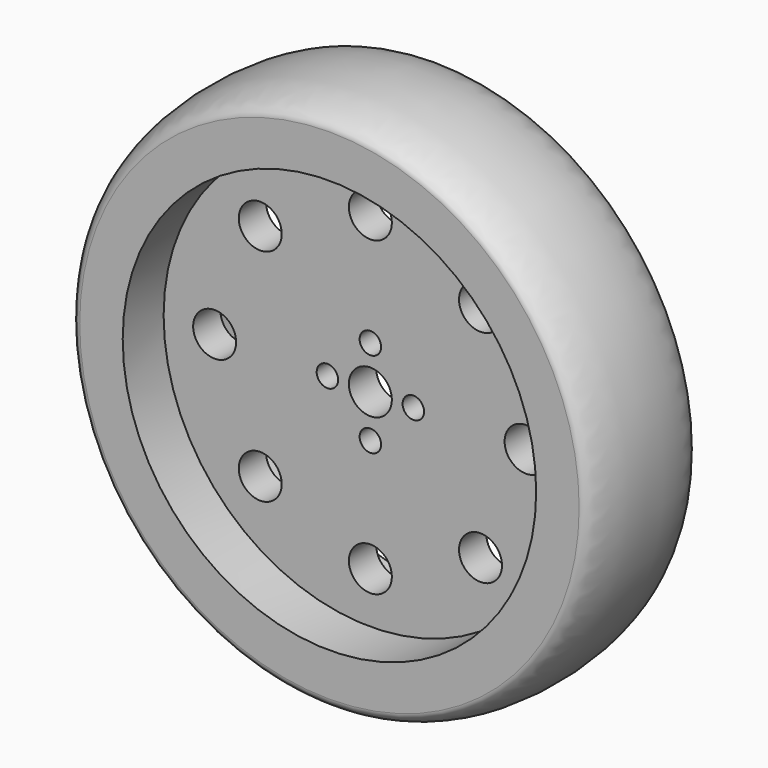
from build123d import *

# Parameters (mm, degrees)
F2_R     = 46.5
F2_R_2   = 38.5
F3_DEPTH = 12.7
F2_R_3   = 4
F2_R_4   = 2
F4_DEPTH = 3.175


# Not quite as in the source:
# - a length typed as a fraction of an inch, garbled in the dataset ("3 / 203.2 mm" for 3/8 in), is restored


with BuildPart() as f1:
    # F0 (on Right) → F1 (revolve)
    with BuildSketch(Plane.YZ):
        with BuildLine():
            Line((-12.7, 46.5), (12.7, 46.5))
            add(Edge.make_bspline(
                [(12.7, 46.5), (12.7, 50.2635093224), (0, 50.2635093224), (-12.7, 50.2635093224), (-12.7, 46.5)],
                knots=[0, 0, 0, 1.5707963268, 1.5707963268, 3.1415926536, 3.1415926536, 3.1415926536], degree=2, weights=[1, 0.7071067812, 1, 0.7071067812, 1]))
        make_face()
    revolve(axis=Axis((0, 0, 0), (0, 1, 0)))

    # F2 (on Front) → F3 (join, symmetric)
    with BuildSketch(Plane.XZ):
        Circle(F2_R)
        Circle(F2_R_2, mode=Mode.SUBTRACT)
    extrude(amount=F3_DEPTH, both=True)

    # F2 (on Front) → F4 (join, symmetric)
    with BuildSketch(Plane.XZ):
        Circle(F2_R_2)
        with Locations((-20.5060966544, -20.5060966544)):
            Circle(F2_R_3, mode=Mode.SUBTRACT)
        with Locations((0, -29)):
            Circle(F2_R_3, mode=Mode.SUBTRACT)
        with Locations((20.5060966544, -20.5060966544)):
            Circle(F2_R_3, mode=Mode.SUBTRACT)
        with Locations((0, -8)):
            Circle(F2_R_4, mode=Mode.SUBTRACT)
        with Locations((-29, 0)):
            Circle(F2_R_3, mode=Mode.SUBTRACT)
        with Locations((-8, 0)):
            Circle(F2_R_4, mode=Mode.SUBTRACT)
        with Locations((-20.5060966544, 20.5060966544)):
            Circle(F2_R_3, mode=Mode.SUBTRACT)
        Circle(F2_R_3, mode=Mode.SUBTRACT)
        with Locations((8, 0)):
            Circle(F2_R_4, mode=Mode.SUBTRACT)
        with Locations((0, 8)):
            Circle(F2_R_4, mode=Mode.SUBTRACT)
        with Locations((20.5060966544, 20.5060966544)):
            Circle(F2_R_3, mode=Mode.SUBTRACT)
        with Locations((29, 0)):
            Circle(F2_R_3, mode=Mode.SUBTRACT)
        with Locations((0, 29)):
            Circle(F2_R_3, mode=Mode.SUBTRACT)
    extrude(amount=F4_DEPTH, both=True)


solid = f1.part
